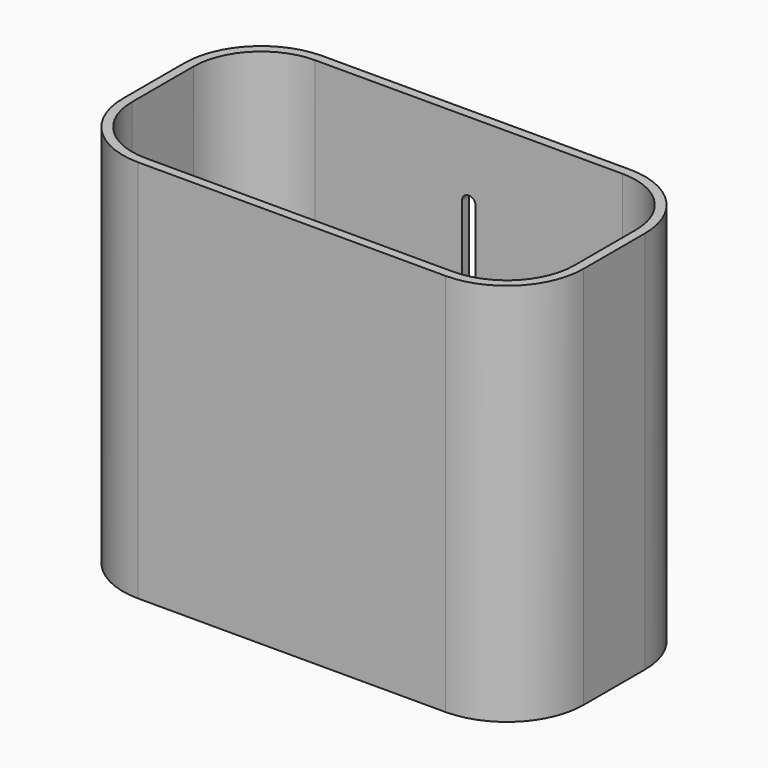
from build123d import *

# Parameters (mm, degrees)
F0_W     = 76.2
F0_H     = 38.1
F1_DEPTH = 63.5
F2_R     = 12.7
F3_T     = -1.524
F4_W     = 2.286
F4_H     = 40.64
F5_DEPTH = 1.524
F6_R     = 1.14299


# Not quite as in the source:
# - a fillet or chamfer is up to 0.001 mm smaller than in the source, because OpenCascade refuses the exact size


with BuildPart() as f1:
    # F0 (on Top) → F1 (new body)
    with BuildSketch(Plane.XY):
        Rectangle(F0_W, F0_H)
    extrude(amount=F1_DEPTH)

    # F2
    f2_edges = [f1.edges().sort_by_distance(p)[0] for p in [
        (38.1, -19.05, 31.75),
        (38.1, 19.05, 31.75),
        (-38.1, -19.05, 31.75),
        (-38.1, 19.05, 31.75),
    ]]
    fillet(f2_edges, radius=F2_R)

    # F3
    f3_openings = [f1.faces().sort_by_distance(p)[0] for p in [
        (0, 0, 63.5),
    ]]
    offset(amount=F3_T, openings=f3_openings)

    # F4 (on face) → F5 (cut, through all)
    with BuildSketch(Plane(origin=(0, 19.05, 0), x_dir=(-1, 0, 0), z_dir=(0, 1, 0))):
        with Locations((0, 31.75)):
            Rectangle(F4_W, F4_H)
    extrude(amount=-F5_DEPTH, mode=Mode.SUBTRACT)

    # F6 (radius 1.143 in the source; OpenCascade refuses exactly that, so slightly less here)
    f6_edges = [f1.edges().sort_by_distance(p)[0] for p in [
        (1.143, 18.288, 52.07),
        (-1.143, 18.288, 52.07),
        (1.143, 18.288, 11.43),
        (-1.143, 18.288, 11.43),
    ]]
    fillet(f6_edges, radius=F6_R)


solid = f1.part
